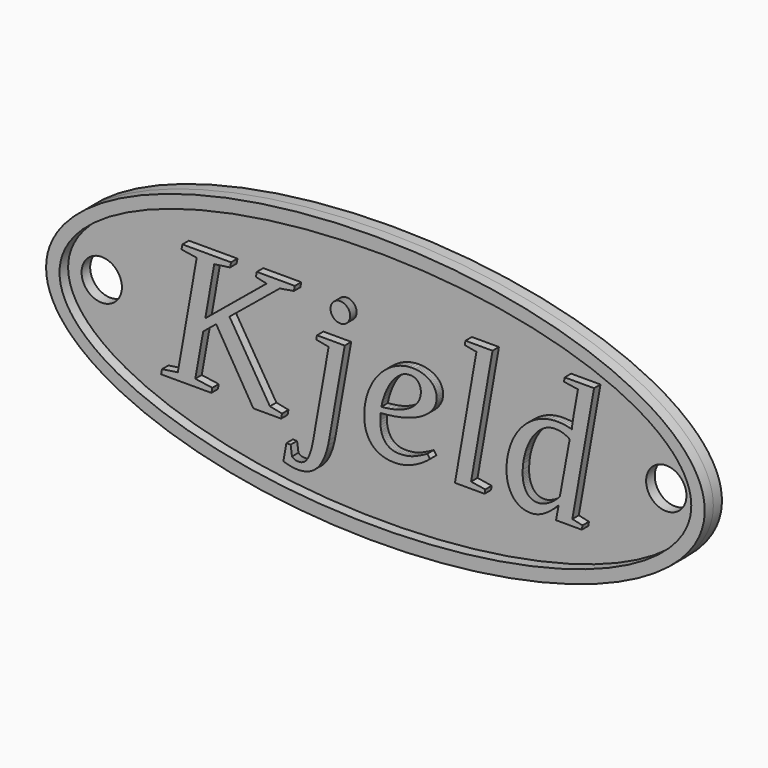
from build123d import *

# Parameters (mm, degrees)
F0_R     = 3
F1_DEPTH = 1.6
F2_DEPTH = 1.6
F3_DEPTH = 1.2


# Not quite as in the source:
# - a feature names something its author has since deleted; it is built from what else it names


with BuildPart() as f1:
    # F0 (on Front) → F1 (new body)
    with BuildSketch(Plane.XZ):
        with BuildLine():
            add(Edge.make_bspline(
                [(49, 0), (49, 34.6410161514), (-24.5, 17.3205080757), (-98, 0), (-24.5, -17.3205080757), (49, -34.6410161514), (49, 0)],
                knots=[0, 0, 0, 2.0943951024, 2.0943951024, 4.1887902048, 4.1887902048, 6.2831853072, 6.2831853072, 6.2831853072], degree=2, weights=[1, 0.5, 1, 0.5, 1, 0.5, 1]))
        make_face()
        with BuildLine():
            add(Edge.make_bspline(
                [(47, 0), (47, 31.1769145362), (-23.5, 15.5884572681), (-94, 0), (-23.5, -15.5884572681), (47, -31.1769145362), (47, 0)],
                knots=[0, 0, 0, 2.0943951024, 2.0943951024, 4.1887902048, 4.1887902048, 6.2831853072, 6.2831853072, 6.2831853072], degree=2, weights=[1, 0.5, 1, 0.5, 1, 0.5, 1]))
        make_face(mode=Mode.SUBTRACT)
        with BuildLine():
            add(Edge.make_bspline(
                [(47, 0), (47, 31.1769145362), (-23.5, 15.5884572681), (-94, 0), (-23.5, -15.5884572681), (47, -31.1769145362), (47, 0)],
                knots=[0, 0, 0, 2.0943951024, 2.0943951024, 4.1887902048, 4.1887902048, 6.2831853072, 6.2831853072, 6.2831853072], degree=2, weights=[1, 0.5, 1, 0.5, 1, 0.5, 1]))
        make_face()
        Polygon((-4.88085, 3.9466265909), (-7.22335, -9.2331734091), (-7.36215, -9.9206734091), (-7.52285, -10.5558734091), (-7.61145, -10.8539734091), (-7.70545, -11.1389734091), (-7.80495, -11.4109734091), (-7.90995, -11.6699734091), (-8.01705, -11.9198734091), (-8.12955, -12.1579734091), (-8.24755, -12.3842734091), (-8.37105, -12.5988734091), (-8.49995, -12.8016734091), (-8.63435, -12.9926734091), (-8.77425, -13.1718734091), (-8.91965, -13.3392734091), (-9.06685, -13.4953734091), (-9.21915, -13.6405734091), (-9.37655, -13.7747734091), (-9.53895, -13.8979734091), (-9.70635, -14.0103734091), (-9.87885, -14.1116734091), (-10.05635, -14.2021734091), (-10.23895, -14.2816734091), (-10.42615, -14.3510734091), (-10.61755, -14.4112734091), (-10.81325, -14.4621734091), (-11.01305, -14.5037734091), (-11.21705, -14.5361734091), (-11.42535, -14.5593734091), (-11.63785, -14.5732734091), (-11.85445, -14.5778734091), (-12.15565, -14.5694734091), (-12.45355, -14.5441734091), (-12.74805, -14.5021734091), (-13.03915, -14.4432734091), (-13.31685, -14.3809734091), (-13.44685, -14.3485734091), (-13.57095, -14.3153734091), (-13.68915, -14.2812734091), (-13.80145, -14.2463734091), (-13.90795, -14.2105734091), (-14.00845, -14.1739734091), (-13.56425, -11.6564734091), (-12.93145, -11.6564734091), (-12.72955, -13.1373734091), (-12.69125, -13.1737734091), (-12.65045, -13.2088734091), (-12.60715, -13.2427734091), (-12.56125, -13.2753734091), (-12.51285, -13.3066734091), (-12.46195, -13.3367734091), (-12.40855, -13.3655734091), (-12.35255, -13.3931734091), (-12.29345, -13.4183734091), (-12.23055, -13.4402734091), (-12.16385, -13.4587734091), (-12.09345, -13.4739734091), (-12.01915, -13.4856734091), (-11.94115, -13.4940734091), (-11.85935, -13.4991734091), (-11.77365, -13.5008734091), (-11.68025, -13.4983734091), (-11.58855, -13.4907734091), (-11.49855, -13.4781734091), (-11.41025, -13.4604734091), (-11.32355, -13.4377734091), (-11.23855, -13.4099734091), (-11.15525, -13.3771734091), (-11.07365, -13.3392734091), (-10.99375, -13.2951734091), (-10.91545, -13.2433734091), (-10.83885, -13.1840734091), (-10.76395, -13.1171734091), (-10.69075, -13.0426734091), (-10.61925, -12.9606734091), (-10.54945, -12.8710734091), (-10.48125, -12.7738734091), (-10.41465, -12.6682734091), (-10.34915, -12.5533734091), (-10.28505, -12.4292734091), (-10.22215, -12.2959734091), (-10.16045, -12.1533734091), (-10.10015, -12.0014734091), (-10.04105, -11.8403734091), (-9.98315, -11.6699734091), (-9.92655, -11.4923734091), (-9.87125, -11.3030734091), (-9.81725, -11.1019734091), (-9.76445, -10.8890734091), (-9.71285, -10.6644734091), (-9.66255, -10.4279734091), (-9.61355, -10.1797734091), (-9.56585, -9.9197734091), (-7.27715, 3.0042265909), (-9.12155, 3.3408265909), (-9.01385, 3.9466265909), align=None, mode=Mode.SUBTRACT)
        Polygon((8.79375, 1.6700265909), (8.79775, 1.5234265909), (8.78915, 1.3061265909), (8.76325, 1.0917265909), (8.72015, 0.8803265909), (8.65985, 0.6718265909), (8.58215, 0.4663265909), (8.48735, 0.2638265909), (8.37515, 0.0641265909), (8.24585, -0.1324734091), (8.09985, -0.3253734091), (7.93785, -0.5136734091), (7.75995, -0.6972734091), (7.56595, -0.8762734091), (7.35605, -1.0506734091), (7.13015, -1.2204734091), (6.88825, -1.3855734091), (6.63035, -1.5460734091), (6.35985, -1.6979734091), (6.07335, -1.8439734091), (5.77085, -1.9840734091), (5.45235, -2.1182734091), (5.11785, -2.2465734091), (4.76745, -2.3689734091), (4.01855, -2.5961734091), (3.21585, -2.7871734091), (2.35595, -2.9428734091), (1.43885, -3.0631734091), (0.46445, -3.1481734091), (0.46275, -3.1637734091), (0.46085, -3.1805734091), (0.45895, -3.1982734091), (0.45685, -3.2171734091), (0.45475, -3.2369734091), (0.45245, -3.2579734091), (0.45015, -3.2798734091), (0.44765, -3.3029734091), (0.44235, -3.3521734091), (0.43665, -3.4055734091), (0.43055, -3.4632734091), (0.42405, -3.5250734091), (0.42095, -3.5904734091), (0.41585, -3.7301734091), (0.41255, -3.8816734091), (0.41085, -4.0448734091), (0.41065, -4.1308734091), (0.41815, -4.4581734091), (0.44095, -4.7804734091), (0.47875, -5.0976734091), (0.53175, -5.4098734091), (0.56835, -5.5625734091), (0.61085, -5.7110734091), (0.65925, -5.8553734091), (0.71355, -5.9954734091), (0.77365, -6.1313734091), (0.83975, -6.2630734091), (0.91165, -6.3904734091), (0.98955, -6.5137734091), (1.07385, -6.6319734091), (1.16535, -6.7442734091), (1.26405, -6.8507734091), (1.36985, -6.9512734091), (1.48275, -7.0459734091), (1.60285, -7.1347734091), (1.73015, -7.2175734091), (1.86455, -7.2945734091), (2.00715, -7.3608734091), (2.15905, -7.4182734091), (2.32015, -7.4668734091), (2.49055, -7.5066734091), (2.67025, -7.5375734091), (2.85915, -7.5596734091), (3.05725, -7.5728734091), (3.26465, -7.5772734091), (3.56465, -7.5709734091), (3.85875, -7.5520734091), (4.14685, -7.5204734091), (4.42915, -7.4763734091), (4.70555, -7.4195734091), (4.97615, -7.3501734091), (5.24075, -7.2680734091), (5.49945, -7.1734734091), (6.00265, -6.9580734091), (6.95845, -6.4868734091), (7.41115, -6.2310734091), (7.80155, -6.7964734091), (7.57695, -6.9798734091), (7.33375, -7.1666734091), (7.07205, -7.3568734091), (6.79185, -7.5503734091), (6.49565, -7.7413734091), (6.18605, -7.9239734091), (5.52635, -8.2638734091), (5.18475, -8.4119734091), (4.83305, -8.5465734091), (4.47125, -8.6677734091), (4.09935, -8.7754734091), (3.72075, -8.8638734091), (3.33875, -8.9269734091), (2.95335, -8.9647734091), (2.56465, -8.9774734091), (2.28315, -8.9723734091), (2.01095, -8.9572734091), (1.74805, -8.9319734091), (1.49435, -8.8966734091), (1.24995, -8.8511734091), (1.01475, -8.7956734091), (0.78885, -8.7300734091), (0.57215, -8.6543734091), (0.36455, -8.5659734091), (0.16575, -8.4691734091), (-0.02415, -8.3640734091), (-0.20535, -8.2504734091), (-0.37755, -8.1284734091), (-0.54105, -7.9980734091), (-0.69565, -7.8591734091), (-0.84145, -7.7119734091), (-0.97835, -7.5562734091), (-1.10645, -7.3921734091), (-1.22575, -7.2196734091), (-1.33615, -7.0387734091), (-1.43775, -6.8494734091), (-1.53055, -6.6517734091), (-1.61445, -6.4455734091), (-1.68955, -6.2310734091), (-1.75585, -6.0089734091), (-1.81325, -5.7800734091), (-1.86185, -5.5444734091), (-1.90155, -5.3021734091), (-1.93255, -5.0530734091), (-1.96785, -4.5347734091), (-1.97225, -4.2654734091), (-1.95545, -3.6731734091), (-1.90495, -3.0942734091), (-1.82085, -2.5288734091), (-1.70305, -1.9768734091), (-1.55495, -1.4349734091), (-1.37995, -0.9133734091), (-1.17795, -0.4118734091), (-0.94915, 0.0694265909), (-0.69505, 0.5355265909), (-0.41735, 0.9781265909), (-0.11615, 1.3971265909), (0.20865, 1.7926265909), (0.55195, 2.1687265909), (0.90875, 2.5162265909), (1.27895, 2.8351265909), (1.66265, 3.1254265909), (2.06485, 3.3854265909), (2.47715, 3.6134265909), (2.89955, 3.8095265909), (3.33195, 3.9735265909), (3.77795, 4.1090265909), (4.22725, 4.2058265909), (4.67995, 4.2638265909), (5.13595, 4.2832265909), (5.55495, 4.2697265909), (5.75565, 4.2529265909), (5.95045, 4.2293265909), (6.13935, 4.1990265909), (6.32235, 4.1620265909), (6.49945, 4.1183265909), (6.67075, 4.0678265909), (6.83895, 4.0146265909), (7.00055, 3.9559265909), (7.15535, 3.8917265909), (7.30345, 3.8221265909), (7.44485, 3.7470265909), (7.57945, 3.6664265909), (7.70735, 3.5804265909), (7.82845, 3.4889265909), (7.94275, 3.3957265909), (8.04975, 3.2979265909), (8.14965, 3.1955265909), (8.24245, 3.0884265909), (8.32805, 2.9767265909), (8.40655, 2.8604265909), (8.47785, 2.7394265909), (8.54205, 2.6138265909), (8.60195, 2.4878265909), (8.65395, 2.3589265909), (8.69785, 2.2270265909), (8.73385, 2.0922265909), (8.76185, 1.9544265909), (8.78185, 1.8136265909), align=None, mode=Mode.SUBTRACT)
        with Locations((-42, 0)):
            Circle(F0_R, mode=Mode.SUBTRACT)
        Polygon((-17.96715, 9.3451265909), (-12.31285, 9.3451265909), (-12.44745, 8.6316265909), (-14.54765, 8.2816265909), (-22.03285, 2.1561265909), (-16.01505, -7.6311734091), (-14.21105, -7.9946734091), (-14.34575, -8.7081734091), (-18.47875, -8.7081734091), (-24.01185, 0.5271265909), (-25.93695, -1.0479734091), (-27.12165, -7.6311734091), (-24.59075, -7.9946734091), (-24.72535, -8.7081734091), (-32.21055, -8.7081734091), (-32.07595, -7.9946734091), (-29.71995, -7.6311734091), (-26.90625, 8.2816265909), (-29.16805, 8.6316265909), (-29.03335, 9.3451265909), (-21.80395, 9.3451265909), (-21.93865, 8.6316265909), (-24.30805, 8.2816265909), (-25.62735, 0.7695265909), (-16.49975, 8.2816265909), (-18.10175, 8.6316265909), align=None, mode=Mode.SUBTRACT)
        Polygon((-4.07495, 8.1533265909), (-4.07305, 8.0796265909), (-4.07495, 8.0060265909), (-4.08065, 7.9332265909), (-4.09015, 7.8613265909), (-4.10335, 7.7902265909), (-4.12045, 7.7199265909), (-4.14125, 7.6505265909), (-4.16585, 7.5819265909), (-4.19425, 7.5142265909), (-4.22265, 7.4511265909), (-4.25405, 7.3897265909), (-4.28825, 7.3299265909), (-4.32555, 7.2719265909), (-4.36575, 7.2155265909), (-4.40885, 7.1608265909), (-4.45485, 7.1078265909), (-4.50395, 7.0565265909), (-4.55545, 7.0073265909), (-4.60905, 6.9606265909), (-4.66485, 6.9164265909), (-4.72265, 6.8747265909), (-4.78265, 6.8356265909), (-4.84465, 6.7990265909), (-4.90885, 6.7649265909), (-4.97505, 6.7334265909), (-5.04285, 6.7081265909), (-5.11145, 6.6863265909), (-5.18085, 6.6677265909), (-5.25105, 6.6526265909), (-5.32215, 6.6408265909), (-5.39415, 6.6324265909), (-5.46685, 6.6274265909), (-5.54055, 6.6257265909), (-5.61415, 6.6274265909), (-5.68695, 6.6324265909), (-5.75885, 6.6408265909), (-5.82995, 6.6526265909), (-5.90025, 6.6677265909), (-5.96965, 6.6863265909), (-6.03825, 6.7081265909), (-6.10595, 6.7334265909), (-6.23045, 6.7990265909), (-6.34825, 6.8747265909), (-6.45935, 6.9606265909), (-6.56365, 7.0565265909), (-6.65955, 7.1608265909), (-6.74545, 7.2719265909), (-6.82115, 7.3897265909), (-6.88675, 7.5142265909), (-6.91205, 7.5819265909), (-6.93385, 7.6505265909), (-6.95245, 7.7199265909), (-6.96755, 7.7902265909), (-6.97935, 7.8613265909), (-6.98775, 7.9332265909), (-6.99275, 8.0060265909), (-6.99445, 8.0796265909), (-6.99275, 8.1533265909), (-6.98775, 8.2260265909), (-6.97935, 8.2980265909), (-6.96755, 8.3691265909), (-6.95245, 8.4393265909), (-6.93385, 8.5087265909), (-6.91205, 8.5773265909), (-6.88675, 8.6451265909), (-6.85525, 8.7113265909), (-6.82115, 8.7755265909), (-6.78455, 8.8375265909), (-6.74545, 8.8975265909), (-6.70375, 8.9553265909), (-6.65955, 9.0111265909), (-6.61285, 9.0647265909), (-6.56365, 9.1162265909), (-6.51235, 9.1653265909), (-6.45935, 9.2113265909), (-6.40465, 9.2544265909), (-6.34825, 9.2946265909), (-6.29025, 9.3319265909), (-6.23045, 9.3661265909), (-6.16905, 9.3975265909), (-6.10595, 9.4259265909), (-6.03825, 9.4543265909), (-5.96965, 9.4789265909), (-5.90025, 9.4997265909), (-5.82995, 9.5168265909), (-5.75885, 9.5300265909), (-5.68695, 9.5395265909), (-5.61415, 9.5452265909), (-5.54055, 9.5470265909), (-5.46685, 9.5452265909), (-5.39415, 9.5395265909), (-5.32215, 9.5300265909), (-5.25105, 9.5168265909), (-5.18085, 9.4997265909), (-5.11145, 9.4789265909), (-5.04285, 9.4543265909), (-4.97505, 9.4259265909), (-4.90885, 9.3975265909), (-4.84465, 9.3661265909), (-4.78265, 9.3319265909), (-4.72265, 9.2946265909), (-4.66485, 9.2544265909), (-4.60905, 9.2113265909), (-4.55545, 9.1653265909), (-4.50395, 9.1162265909), (-4.45485, 9.0647265909), (-4.40885, 9.0111265909), (-4.36575, 8.9553265909), (-4.32555, 8.8975265909), (-4.28825, 8.8375265909), (-4.25405, 8.7755265909), (-4.22265, 8.7113265909), (-4.19425, 8.6451265909), (-4.16585, 8.5773265909), (-4.14125, 8.5087265909), (-4.12045, 8.4393265909), (-4.10335, 8.3691265909), (-4.09015, 8.2980265909), (-4.08065, 8.2260265909), align=None, mode=Mode.SUBTRACT)
        Polygon((17.10485, 10.4221265909), (13.91425, -7.7657734091), (16.02785, -8.1023734091), (15.92015, -8.7081734091), (11.51795, -8.7081734091), (14.70855, 9.4932265909), (12.97185, 9.8163265909), (13.07955, 10.4221265909), align=None, mode=Mode.SUBTRACT)
        Polygon((28.66405, 4.0299265909), (28.89875, 3.9601265909), (28.90055, 3.9808265909), (28.90255, 4.0026265909), (28.90475, 4.0254265909), (28.90715, 4.0493265909), (28.91265, 4.1002265909), (28.91895, 4.1553265909), (28.92615, 4.2146265909), (28.93415, 4.2781265909), (28.94295, 4.3459265909), (28.95265, 4.4178265909), (28.97365, 4.5735265909), (29.02075, 4.8898265909), (29.04685, 5.0505265909), (29.07295, 5.2171265909), (29.12005, 5.5403265909), (29.14105, 5.6968265909), (29.15435, 5.7725265909), (29.16715, 5.8448265909), (29.17955, 5.9138265909), (29.19155, 5.9795265909), (29.20315, 6.0417265909), (29.21425, 6.1006265909), (29.22505, 6.1562265909), (29.23535, 6.2083265909), (29.81425, 9.4932265909), (27.74095, 9.8163265909), (27.84865, 10.4221265909), (32.21055, 10.4221265909), (28.97955, -7.7657734091), (30.50085, -8.1023734091), (30.39315, -8.7081734091), (26.55625, -8.7081734091), (26.94665, -6.6079734091), (26.66545, -6.8951734091), (26.38715, -7.1641734091), (26.11175, -7.4151734091), (25.83935, -7.6479734091), (25.56995, -7.8627734091), (25.30345, -8.0594734091), (25.03985, -8.2380734091), (24.77925, -8.3985734091), (24.52135, -8.5373734091), (24.26595, -8.6576734091), (24.01315, -8.7594734091), (23.76275, -8.8427734091), (23.51495, -8.9075734091), (23.26975, -8.9538734091), (23.02695, -8.9816734091), (22.78675, -8.9908734091), (22.58715, -8.9860734091), (22.39215, -8.9715734091), (22.20175, -8.9473734091), (22.01605, -8.9134734091), (21.83495, -8.8699734091), (21.65845, -8.8166734091), (21.48655, -8.7537734091), (21.31935, -8.6812734091), (21.15735, -8.5996734091), (21.00125, -8.5095734091), (20.85105, -8.4111734091), (20.70675, -8.3042734091), (20.56835, -8.1889734091), (20.43585, -8.0653734091), (20.30925, -7.9332734091), (20.18845, -7.7926734091), (20.07385, -7.6406734091), (19.96555, -7.4805734091), (19.86345, -7.3124734091), (19.76775, -7.1363734091), (19.67835, -6.9523734091), (19.59525, -6.7602734091), (19.51855, -6.5602734091), (19.44805, -6.3521734091), (19.38805, -6.1367734091), (19.33615, -5.9146734091), (19.29215, -5.6858734091), (19.22825, -5.2078734091), (19.19625, -4.7030734091), (19.19225, -4.4405734091), (19.20825, -3.8658734091), (19.25615, -3.2995734091), (19.33615, -2.7417734091), (19.44805, -2.1922734091), (19.58935, -1.6487734091), (19.75765, -1.1219734091), (19.95285, -0.6120734091), (20.17505, -0.1190734091), (20.42235, 0.3546265909), (20.69335, 0.8065265909), (20.98785, 1.2364265909), (21.30585, 1.6445265909), (21.65255, 2.0341265909), (22.01935, 2.3951265909), (22.40645, 2.7274265909), (22.81365, 3.0312265909), (23.23945, 3.3105265909), (23.68205, 3.5562265909), (24.14145, 3.7682265909), (24.61765, 3.9466265909), (25.11495, 4.0880265909), (25.62395, 4.1889265909), (26.14485, 4.2495265909), (26.67745, 4.2697265909), (27.00555, 4.2647265909), (27.31695, 4.2495265909), (27.61145, 4.2243265909), (27.88905, 4.1889265909), (28.15915, 4.1443265909), (28.41745, 4.0913265909), align=None, mode=Mode.SUBTRACT)
        with Locations((42, 0)):
            Circle(F0_R, mode=Mode.SUBTRACT)
        Polygon((28.90055, 3.9808265909), (28.89875, 3.9601265909), (28.66405, 4.0299265909), (28.41745, 4.0913265909), (28.15915, 4.1443265909), (27.88905, 4.1889265909), (27.61145, 4.2243265909), (27.31695, 4.2495265909), (27.00555, 4.2647265909), (26.67745, 4.2697265909), (26.14485, 4.2495265909), (25.62395, 4.1889265909), (25.11495, 4.0880265909), (24.61765, 3.9466265909), (24.14145, 3.7682265909), (23.68205, 3.5562265909), (23.23945, 3.3105265909), (22.81365, 3.0312265909), (22.40645, 2.7274265909), (22.01935, 2.3951265909), (21.65255, 2.0341265909), (21.30585, 1.6445265909), (20.98785, 1.2364265909), (20.69335, 0.8065265909), (20.42235, 0.3546265909), (20.17505, -0.1190734091), (19.95285, -0.6120734091), (19.75765, -1.1219734091), (19.58935, -1.6487734091), (19.44805, -2.1922734091), (19.33615, -2.7417734091), (19.25615, -3.2995734091), (19.20825, -3.8658734091), (19.19225, -4.4405734091), (19.19625, -4.7030734091), (19.22825, -5.2078734091), (19.29215, -5.6858734091), (19.33615, -5.9146734091), (19.38805, -6.1367734091), (19.44805, -6.3521734091), (19.51855, -6.5602734091), (19.59525, -6.7602734091), (19.67835, -6.9523734091), (19.76775, -7.1363734091), (19.86345, -7.3124734091), (19.96555, -7.4805734091), (20.07385, -7.6406734091), (20.18845, -7.7926734091), (20.30925, -7.9332734091), (20.43585, -8.0653734091), (20.56835, -8.1889734091), (20.70675, -8.3042734091), (20.85105, -8.4111734091), (21.00125, -8.5095734091), (21.15735, -8.5996734091), (21.31935, -8.6812734091), (21.48655, -8.7537734091), (21.65845, -8.8166734091), (21.83495, -8.8699734091), (22.01605, -8.9134734091), (22.20175, -8.9473734091), (22.39215, -8.9715734091), (22.58715, -8.9860734091), (22.78675, -8.9908734091), (23.02695, -8.9816734091), (23.26975, -8.9538734091), (23.51495, -8.9075734091), (23.76275, -8.8427734091), (24.01315, -8.7594734091), (24.26595, -8.6576734091), (24.52135, -8.5373734091), (24.77925, -8.3985734091), (25.03985, -8.2380734091), (25.30345, -8.0594734091), (25.56995, -7.8627734091), (25.83935, -7.6479734091), (26.11175, -7.4151734091), (26.38715, -7.1641734091), (26.66545, -6.8951734091), (26.94665, -6.6079734091), (26.55625, -8.7081734091), (30.39315, -8.7081734091), (30.50085, -8.1023734091), (28.97955, -7.7657734091), (32.21055, 10.4221265909), (27.84865, 10.4221265909), (27.74095, 9.8163265909), (29.81425, 9.4932265909), (29.23535, 6.2083265909), (29.22505, 6.1562265909), (29.21425, 6.1006265909), (29.20315, 6.0417265909), (29.19155, 5.9795265909), (29.17955, 5.9138265909), (29.16715, 5.8448265909), (29.15435, 5.7725265909), (29.14105, 5.6968265909), (29.12005, 5.5403265909), (29.07295, 5.2171265909), (29.04685, 5.0505265909), (29.02075, 4.8898265909), (28.97365, 4.5735265909), (28.95265, 4.4178265909), (28.94295, 4.3459265909), (28.93415, 4.2781265909), (28.92615, 4.2146265909), (28.91895, 4.1553265909), (28.91265, 4.1002265909), (28.90715, 4.0493265909), (28.90475, 4.0254265909), (28.90255, 4.0026265909), align=None)
        Polygon((28.35185, 2.7064265909), (28.58915, 2.5600265909), (27.12175, -5.4367734091), (26.91535, -5.6527734091), (26.49635, -6.0482734091), (26.28365, -6.2276734091), (26.06885, -6.3949734091), (25.85205, -6.5499734091), (25.63305, -6.6927734091), (25.41195, -6.8233734091), (25.19505, -6.9369734091), (24.98195, -7.0354734091), (24.77265, -7.1187734091), (24.56715, -7.1868734091), (24.36545, -7.2398734091), (24.16755, -7.2777734091), (23.97335, -7.3004734091), (23.78295, -7.3080734091), (23.67885, -7.3053734091), (23.57515, -7.2971734091), (23.47185, -7.2834734091), (23.36905, -7.2642734091), (23.26655, -7.2396734091), (23.16455, -7.2095734091), (23.06295, -7.1740734091), (22.96175, -7.1330734091), (22.86545, -7.0861734091), (22.77165, -7.0329734091), (22.68035, -6.9733734091), (22.59155, -6.9075734091), (22.50535, -6.8353734091), (22.42155, -6.7569734091), (22.34035, -6.6721734091), (22.26175, -6.5810734091), (22.18935, -6.4803734091), (22.12035, -6.3732734091), (22.05475, -6.2598734091), (21.99245, -6.1401734091), (21.93355, -6.0141734091), (21.87805, -5.8818734091), (21.82585, -5.7432734091), (21.77705, -5.5982734091), (21.73285, -5.4430734091), (21.69465, -5.2802734091), (21.66225, -5.1098734091), (21.63575, -4.9318734091), (21.61505, -4.7463734091), (21.60035, -4.5532734091), (21.59155, -4.3525734091), (21.58855, -4.1443734091), (21.59785, -3.7126734091), (21.67185, -2.8443734091), (21.73665, -2.4076734091), (21.82585, -1.9734734091), (22.05475, -1.1253734091), (22.19435, -0.7113734091), (22.35005, -0.3075734091), (22.52085, 0.0829265909), (22.70685, 0.4598265909), (22.90795, 0.8233265909), (23.13005, 1.1683265909), (23.36565, 1.4897265909), (23.61475, 1.7876265909), (23.87725, 2.0619265909), (24.01335, 2.1929265909), (24.29435, 2.4336265909), (24.58715, 2.6456265909), (24.89175, 2.8290265909), (25.04845, 2.9100265909), (25.20815, 2.9826265909), (25.37075, 3.0455265909), (25.53625, 3.0987265909), (25.70475, 3.1422265909), (25.87625, 3.1761265909), (26.05055, 3.2003265909), (26.22795, 3.2148265909), (26.40815, 3.2196265909), (26.58315, 3.2169265909), (26.75145, 3.2087265909), (26.91305, 3.1950265909), (27.06785, 3.1759265909), (27.21595, 3.1513265909), (27.35725, 3.1212265909), (27.49195, 3.0856265909), (27.61985, 3.0446265909), (27.86715, 2.9487265909), (28.11125, 2.8360265909), align=None, mode=Mode.SUBTRACT)
        Polygon((-12.44745, 8.6316265909), (-12.31285, 9.3451265909), (-17.96715, 9.3451265909), (-18.10175, 8.6316265909), (-16.49975, 8.2816265909), (-25.62735, 0.7695265909), (-24.30805, 8.2816265909), (-21.93865, 8.6316265909), (-21.80395, 9.3451265909), (-29.03335, 9.3451265909), (-29.16805, 8.6316265909), (-26.90625, 8.2816265909), (-29.71995, -7.6311734091), (-32.07595, -7.9946734091), (-32.21055, -8.7081734091), (-24.72535, -8.7081734091), (-24.59075, -7.9946734091), (-27.12165, -7.6311734091), (-25.93695, -1.0479734091), (-24.01185, 0.5271265909), (-18.47875, -8.7081734091), (-14.34575, -8.7081734091), (-14.21105, -7.9946734091), (-16.01505, -7.6311734091), (-22.03285, 2.1561265909), (-14.54765, 8.2816265909), align=None)
        Polygon((8.78915, 1.3061265909), (8.79775, 1.5234265909), (8.79375, 1.6700265909), (8.78185, 1.8136265909), (8.76185, 1.9544265909), (8.73385, 2.0922265909), (8.69785, 2.2270265909), (8.65395, 2.3589265909), (8.60195, 2.4878265909), (8.54205, 2.6138265909), (8.47785, 2.7394265909), (8.40655, 2.8604265909), (8.32805, 2.9767265909), (8.24245, 3.0884265909), (8.14965, 3.1955265909), (8.04975, 3.2979265909), (7.94275, 3.3957265909), (7.82845, 3.4889265909), (7.70735, 3.5804265909), (7.57945, 3.6664265909), (7.44485, 3.7470265909), (7.30345, 3.8221265909), (7.15535, 3.8917265909), (7.00055, 3.9559265909), (6.83895, 4.0146265909), (6.67075, 4.0678265909), (6.49945, 4.1183265909), (6.32235, 4.1620265909), (6.13935, 4.1990265909), (5.95045, 4.2293265909), (5.75565, 4.2529265909), (5.55495, 4.2697265909), (5.13595, 4.2832265909), (4.67995, 4.2638265909), (4.22725, 4.2058265909), (3.77795, 4.1090265909), (3.33195, 3.9735265909), (2.89955, 3.8095265909), (2.47715, 3.6134265909), (2.06485, 3.3854265909), (1.66265, 3.1254265909), (1.27895, 2.8351265909), (0.90875, 2.5162265909), (0.55195, 2.1687265909), (0.20865, 1.7926265909), (-0.11615, 1.3971265909), (-0.41735, 0.9781265909), (-0.69505, 0.5355265909), (-0.94915, 0.0694265909), (-1.17795, -0.4118734091), (-1.37995, -0.9133734091), (-1.55495, -1.4349734091), (-1.70305, -1.9768734091), (-1.82085, -2.5288734091), (-1.90495, -3.0942734091), (-1.95545, -3.6731734091), (-1.97225, -4.2654734091), (-1.96785, -4.5347734091), (-1.93255, -5.0530734091), (-1.90155, -5.3021734091), (-1.86185, -5.5444734091), (-1.81325, -5.7800734091), (-1.75585, -6.0089734091), (-1.68955, -6.2310734091), (-1.61445, -6.4455734091), (-1.53055, -6.6517734091), (-1.43775, -6.8494734091), (-1.33615, -7.0387734091), (-1.22575, -7.2196734091), (-1.10645, -7.3921734091), (-0.97835, -7.5562734091), (-0.84145, -7.7119734091), (-0.69565, -7.8591734091), (-0.54105, -7.9980734091), (-0.37755, -8.1284734091), (-0.20535, -8.2504734091), (-0.02415, -8.3640734091), (0.16575, -8.4691734091), (0.36455, -8.5659734091), (0.57215, -8.6543734091), (0.78885, -8.7300734091), (1.01475, -8.7956734091), (1.24995, -8.8511734091), (1.49435, -8.8966734091), (1.74805, -8.9319734091), (2.01095, -8.9572734091), (2.28315, -8.9723734091), (2.56465, -8.9774734091), (2.95335, -8.9647734091), (3.33875, -8.9269734091), (3.72075, -8.8638734091), (4.09935, -8.7754734091), (4.47125, -8.6677734091), (4.83305, -8.5465734091), (5.18475, -8.4119734091), (5.52635, -8.2638734091), (6.18605, -7.9239734091), (6.49565, -7.7413734091), (6.79185, -7.5503734091), (7.07205, -7.3568734091), (7.33375, -7.1666734091), (7.57695, -6.9798734091), (7.80155, -6.7964734091), (7.41115, -6.2310734091), (6.95845, -6.4868734091), (6.00265, -6.9580734091), (5.49945, -7.1734734091), (5.24075, -7.2680734091), (4.97615, -7.3501734091), (4.70555, -7.4195734091), (4.42915, -7.4763734091), (4.14685, -7.5204734091), (3.85875, -7.5520734091), (3.56465, -7.5709734091), (3.26465, -7.5772734091), (3.05725, -7.5728734091), (2.85915, -7.5596734091), (2.67025, -7.5375734091), (2.49055, -7.5066734091), (2.32015, -7.4668734091), (2.15905, -7.4182734091), (2.00715, -7.3608734091), (1.86455, -7.2945734091), (1.73015, -7.2175734091), (1.60285, -7.1347734091), (1.48275, -7.0459734091), (1.36985, -6.9512734091), (1.26405, -6.8507734091), (1.16535, -6.7442734091), (1.07385, -6.6319734091), (0.98955, -6.5137734091), (0.91165, -6.3904734091), (0.83975, -6.2630734091), (0.77365, -6.1313734091), (0.71355, -5.9954734091), (0.65925, -5.8553734091), (0.61085, -5.7110734091), (0.56835, -5.5625734091), (0.53175, -5.4098734091), (0.47875, -5.0976734091), (0.44095, -4.7804734091), (0.41815, -4.4581734091), (0.41065, -4.1308734091), (0.41085, -4.0448734091), (0.41255, -3.8816734091), (0.41585, -3.7301734091), (0.42095, -3.5904734091), (0.42405, -3.5250734091), (0.43055, -3.4632734091), (0.43665, -3.4055734091), (0.44235, -3.3521734091), (0.44765, -3.3029734091), (0.45015, -3.2798734091), (0.45245, -3.2579734091), (0.45475, -3.2369734091), (0.45685, -3.2171734091), (0.45895, -3.1982734091), (0.46085, -3.1805734091), (0.46275, -3.1637734091), (0.46445, -3.1481734091), (1.43885, -3.0631734091), (2.35595, -2.9428734091), (3.21585, -2.7871734091), (4.01855, -2.5961734091), (4.76745, -2.3689734091), (5.11785, -2.2465734091), (5.45235, -2.1182734091), (5.77085, -1.9840734091), (6.07335, -1.8439734091), (6.35985, -1.6979734091), (6.63035, -1.5460734091), (6.88825, -1.3855734091), (7.13015, -1.2204734091), (7.35605, -1.0506734091), (7.56595, -0.8762734091), (7.75995, -0.6972734091), (7.93785, -0.5136734091), (8.09985, -0.3253734091), (8.24585, -0.1324734091), (8.37515, 0.0641265909), (8.48735, 0.2638265909), (8.58215, 0.4663265909), (8.65985, 0.6718265909), (8.72015, 0.8803265909), (8.76325, 1.0917265909), align=None)
        Polygon((1.28315, -2.2309734091), (0.57215, -2.2999734091), (0.67315, -1.8144734091), (0.80105, -1.3272734091), (0.95585, -0.8384734091), (1.13755, -0.3478734091), (1.34285, 0.1376265909), (1.56835, 0.5978265909), (1.81405, 1.0328265909), (2.07995, 1.4426265909), (2.22345, 1.6365265909), (2.52295, 1.9966265909), (2.67905, 2.1628265909), (2.83935, 2.3198265909), (3.00385, 2.4674265909), (3.17255, 2.6058265909), (3.34545, 2.7350265909), (3.52195, 2.8549265909), (3.70135, 2.9588265909), (3.88375, 3.0467265909), (4.06905, 3.1187265909), (4.25735, 3.1746265909), (4.44855, 3.2146265909), (4.64265, 3.2386265909), (4.83975, 3.2466265909), (4.93595, 3.2447265909), (5.02915, 3.2390265909), (5.11935, 3.2295265909), (5.20665, 3.2163265909), (5.29105, 3.1992265909), (5.37245, 3.1784265909), (5.45085, 3.1538265909), (5.52635, 3.1254265909), (5.59895, 3.0932265909), (5.66855, 3.0572265909), (5.73525, 3.0175265909), (5.79905, 2.9739265909), (5.85975, 2.9266265909), (5.91765, 2.8755265909), (5.97255, 2.8206265909), (6.02455, 2.7619265909), (6.07505, 2.7003265909), (6.12235, 2.6365265909), (6.16635, 2.5707265909), (6.20705, 2.5028265909), (6.24455, 2.4327265909), (6.27885, 2.3606265909), (6.30975, 2.2863265909), (6.33755, 2.2099265909), (6.36195, 2.1315265909), (6.38315, 2.0509265909), (6.40105, 1.9683265909), (6.41575, 1.8835265909), (6.42715, 1.7966265909), (6.43535, 1.7076265909), (6.44185, 1.5234265909), (6.43615, 1.3523265909), (6.41915, 1.1826265909), (6.39075, 1.0141265909), (6.35095, 0.8469265909), (6.29985, 0.6809265909), (6.23735, 0.5162265909), (6.16355, 0.3527265909), (6.07835, 0.1906265909), (5.98155, 0.0341265909), (5.87305, -0.1190734091), (5.75275, -0.2688734091), (5.62065, -0.4152734091), (5.47675, -0.5582734091), (5.32105, -0.6979734091), (5.15365, -0.8342734091), (4.97445, -0.9671734091), (4.78675, -1.0927734091), (4.58735, -1.2137734091), (4.37615, -1.3300734091), (4.15325, -1.4417734091), (3.91845, -1.5487734091), (3.67195, -1.6512734091), (3.41365, -1.7490734091), (3.14355, -1.8422734091), (2.86185, -1.9259734091), (2.56885, -2.0021734091), (1.94875, -2.1316734091), align=None, mode=Mode.SUBTRACT)
        Polygon((27.12175, -5.4367734091), (28.58915, 2.5600265909), (28.35185, 2.7064265909), (28.11125, 2.8360265909), (27.86715, 2.9487265909), (27.61985, 3.0446265909), (27.49195, 3.0856265909), (27.35725, 3.1212265909), (27.21595, 3.1513265909), (27.06785, 3.1759265909), (26.91305, 3.1950265909), (26.75145, 3.2087265909), (26.58315, 3.2169265909), (26.40815, 3.2196265909), (26.22795, 3.2148265909), (26.05055, 3.2003265909), (25.87625, 3.1761265909), (25.70475, 3.1422265909), (25.53625, 3.0987265909), (25.37075, 3.0455265909), (25.20815, 2.9826265909), (25.04845, 2.9100265909), (24.89175, 2.8290265909), (24.58715, 2.6456265909), (24.29435, 2.4336265909), (24.01335, 2.1929265909), (23.87725, 2.0619265909), (23.61475, 1.7876265909), (23.36565, 1.4897265909), (23.13005, 1.1683265909), (22.90795, 0.8233265909), (22.70685, 0.4598265909), (22.52085, 0.0829265909), (22.35005, -0.3075734091), (22.19435, -0.7113734091), (22.05475, -1.1253734091), (21.82585, -1.9734734091), (21.73665, -2.4076734091), (21.67185, -2.8443734091), (21.59785, -3.7126734091), (21.58855, -4.1443734091), (21.59155, -4.3525734091), (21.60035, -4.5532734091), (21.61505, -4.7463734091), (21.63575, -4.9318734091), (21.66225, -5.1098734091), (21.69465, -5.2802734091), (21.73285, -5.4430734091), (21.77705, -5.5982734091), (21.82585, -5.7432734091), (21.87805, -5.8818734091), (21.93355, -6.0141734091), (21.99245, -6.1401734091), (22.05475, -6.2598734091), (22.12035, -6.3732734091), (22.18935, -6.4803734091), (22.26175, -6.5810734091), (22.34035, -6.6721734091), (22.42155, -6.7569734091), (22.50535, -6.8353734091), (22.59155, -6.9075734091), (22.68035, -6.9733734091), (22.77165, -7.0329734091), (22.86545, -7.0861734091), (22.96175, -7.1330734091), (23.06295, -7.1740734091), (23.16455, -7.2095734091), (23.26655, -7.2396734091), (23.36905, -7.2642734091), (23.47185, -7.2834734091), (23.57515, -7.2971734091), (23.67885, -7.3053734091), (23.78295, -7.3080734091), (23.97335, -7.3004734091), (24.16755, -7.2777734091), (24.36545, -7.2398734091), (24.56715, -7.1868734091), (24.77265, -7.1187734091), (24.98195, -7.0354734091), (25.19505, -6.9369734091), (25.41195, -6.8233734091), (25.63305, -6.6927734091), (25.85205, -6.5499734091), (26.06885, -6.3949734091), (26.28365, -6.2276734091), (26.49635, -6.0482734091), (26.91535, -5.6527734091), align=None)
        Polygon((16.02785, -8.1023734091), (13.91425, -7.7657734091), (17.10485, 10.4221265909), (13.07955, 10.4221265909), (12.97185, 9.8163265909), (14.70855, 9.4932265909), (11.51795, -8.7081734091), (15.92015, -8.7081734091), align=None)
        Polygon((-7.36215, -9.9206734091), (-7.22335, -9.2331734091), (-4.88085, 3.9466265909), (-9.01385, 3.9466265909), (-9.12155, 3.3408265909), (-7.27715, 3.0042265909), (-9.56585, -9.9197734091), (-9.61355, -10.1797734091), (-9.66255, -10.4279734091), (-9.71285, -10.6644734091), (-9.76445, -10.8890734091), (-9.81725, -11.1019734091), (-9.87125, -11.3030734091), (-9.92655, -11.4923734091), (-9.98315, -11.6699734091), (-10.04105, -11.8403734091), (-10.10015, -12.0014734091), (-10.16045, -12.1533734091), (-10.22215, -12.2959734091), (-10.28505, -12.4292734091), (-10.34915, -12.5533734091), (-10.41465, -12.6682734091), (-10.48125, -12.7738734091), (-10.54945, -12.8710734091), (-10.61925, -12.9606734091), (-10.69075, -13.0426734091), (-10.76395, -13.1171734091), (-10.83885, -13.1840734091), (-10.91545, -13.2433734091), (-10.99375, -13.2951734091), (-11.07365, -13.3392734091), (-11.15525, -13.3771734091), (-11.23855, -13.4099734091), (-11.32355, -13.4377734091), (-11.41025, -13.4604734091), (-11.49855, -13.4781734091), (-11.58855, -13.4907734091), (-11.68025, -13.4983734091), (-11.77365, -13.5008734091), (-11.85935, -13.4991734091), (-11.94115, -13.4940734091), (-12.01915, -13.4856734091), (-12.09345, -13.4739734091), (-12.16385, -13.4587734091), (-12.23055, -13.4402734091), (-12.29345, -13.4183734091), (-12.35255, -13.3931734091), (-12.40855, -13.3655734091), (-12.46195, -13.3367734091), (-12.51285, -13.3066734091), (-12.56125, -13.2753734091), (-12.60715, -13.2427734091), (-12.65045, -13.2088734091), (-12.69125, -13.1737734091), (-12.72955, -13.1373734091), (-12.93145, -11.6564734091), (-13.56425, -11.6564734091), (-14.00845, -14.1739734091), (-13.90795, -14.2105734091), (-13.80145, -14.2463734091), (-13.68915, -14.2812734091), (-13.57095, -14.3153734091), (-13.44685, -14.3485734091), (-13.31685, -14.3809734091), (-13.03915, -14.4432734091), (-12.74805, -14.5021734091), (-12.45355, -14.5441734091), (-12.15565, -14.5694734091), (-11.85445, -14.5778734091), (-11.63785, -14.5732734091), (-11.42535, -14.5593734091), (-11.21705, -14.5361734091), (-11.01305, -14.5037734091), (-10.81325, -14.4621734091), (-10.61755, -14.4112734091), (-10.42615, -14.3510734091), (-10.23895, -14.2816734091), (-10.05635, -14.2021734091), (-9.87885, -14.1116734091), (-9.70635, -14.0103734091), (-9.53895, -13.8979734091), (-9.37655, -13.7747734091), (-9.21915, -13.6405734091), (-9.06685, -13.4953734091), (-8.91965, -13.3392734091), (-8.77425, -13.1718734091), (-8.63435, -12.9926734091), (-8.49995, -12.8016734091), (-8.37105, -12.5988734091), (-8.24755, -12.3842734091), (-8.12955, -12.1579734091), (-8.01705, -11.9198734091), (-7.90995, -11.6699734091), (-7.80495, -11.4109734091), (-7.70545, -11.1389734091), (-7.61145, -10.8539734091), (-7.52285, -10.5558734091), align=None)
        Polygon((0.67315, -1.8144734091), (0.57215, -2.2999734091), (1.28315, -2.2309734091), (1.94875, -2.1316734091), (2.56885, -2.0021734091), (2.86185, -1.9259734091), (3.14355, -1.8422734091), (3.41365, -1.7490734091), (3.67195, -1.6512734091), (3.91845, -1.5487734091), (4.15325, -1.4417734091), (4.37615, -1.3300734091), (4.58735, -1.2137734091), (4.78675, -1.0927734091), (4.97445, -0.9671734091), (5.15365, -0.8342734091), (5.32105, -0.6979734091), (5.47675, -0.5582734091), (5.62065, -0.4152734091), (5.75275, -0.2688734091), (5.87305, -0.1190734091), (5.98155, 0.0341265909), (6.07835, 0.1906265909), (6.16355, 0.3527265909), (6.23735, 0.5162265909), (6.29985, 0.6809265909), (6.35095, 0.8469265909), (6.39075, 1.0141265909), (6.41915, 1.1826265909), (6.43615, 1.3523265909), (6.44185, 1.5234265909), (6.43535, 1.7076265909), (6.42715, 1.7966265909), (6.41575, 1.8835265909), (6.40105, 1.9683265909), (6.38315, 2.0509265909), (6.36195, 2.1315265909), (6.33755, 2.2099265909), (6.30975, 2.2863265909), (6.27885, 2.3606265909), (6.24455, 2.4327265909), (6.20705, 2.5028265909), (6.16635, 2.5707265909), (6.12235, 2.6365265909), (6.07505, 2.7003265909), (6.02455, 2.7619265909), (5.97255, 2.8206265909), (5.91765, 2.8755265909), (5.85975, 2.9266265909), (5.79905, 2.9739265909), (5.73525, 3.0175265909), (5.66855, 3.0572265909), (5.59895, 3.0932265909), (5.52635, 3.1254265909), (5.45085, 3.1538265909), (5.37245, 3.1784265909), (5.29105, 3.1992265909), (5.20665, 3.2163265909), (5.11935, 3.2295265909), (5.02915, 3.2390265909), (4.93595, 3.2447265909), (4.83975, 3.2466265909), (4.64265, 3.2386265909), (4.44855, 3.2146265909), (4.25735, 3.1746265909), (4.06905, 3.1187265909), (3.88375, 3.0467265909), (3.70135, 2.9588265909), (3.52195, 2.8549265909), (3.34545, 2.7350265909), (3.17255, 2.6058265909), (3.00385, 2.4674265909), (2.83935, 2.3198265909), (2.67905, 2.1628265909), (2.52295, 1.9966265909), (2.22345, 1.6365265909), (2.07995, 1.4426265909), (1.81405, 1.0328265909), (1.56835, 0.5978265909), (1.34285, 0.1376265909), (1.13755, -0.3478734091), (0.95585, -0.8384734091), (0.80105, -1.3272734091), align=None)
        Polygon((-4.07495, 8.0060265909), (-4.07305, 8.0796265909), (-4.07495, 8.1533265909), (-4.08065, 8.2260265909), (-4.09015, 8.2980265909), (-4.10335, 8.3691265909), (-4.12045, 8.4393265909), (-4.14125, 8.5087265909), (-4.16585, 8.5773265909), (-4.19425, 8.6451265909), (-4.22265, 8.7113265909), (-4.25405, 8.7755265909), (-4.28825, 8.8375265909), (-4.32555, 8.8975265909), (-4.36575, 8.9553265909), (-4.40885, 9.0111265909), (-4.45485, 9.0647265909), (-4.50395, 9.1162265909), (-4.55545, 9.1653265909), (-4.60905, 9.2113265909), (-4.66485, 9.2544265909), (-4.72265, 9.2946265909), (-4.78265, 9.3319265909), (-4.84465, 9.3661265909), (-4.90885, 9.3975265909), (-4.97505, 9.4259265909), (-5.04285, 9.4543265909), (-5.11145, 9.4789265909), (-5.18085, 9.4997265909), (-5.25105, 9.5168265909), (-5.32215, 9.5300265909), (-5.39415, 9.5395265909), (-5.46685, 9.5452265909), (-5.54055, 9.5470265909), (-5.61415, 9.5452265909), (-5.68695, 9.5395265909), (-5.75885, 9.5300265909), (-5.82995, 9.5168265909), (-5.90025, 9.4997265909), (-5.96965, 9.4789265909), (-6.03825, 9.4543265909), (-6.10595, 9.4259265909), (-6.16905, 9.3975265909), (-6.23045, 9.3661265909), (-6.29025, 9.3319265909), (-6.34825, 9.2946265909), (-6.40465, 9.2544265909), (-6.45935, 9.2113265909), (-6.51235, 9.1653265909), (-6.56365, 9.1162265909), (-6.61285, 9.0647265909), (-6.65955, 9.0111265909), (-6.70375, 8.9553265909), (-6.74545, 8.8975265909), (-6.78455, 8.8375265909), (-6.82115, 8.7755265909), (-6.85525, 8.7113265909), (-6.88675, 8.6451265909), (-6.91205, 8.5773265909), (-6.93385, 8.5087265909), (-6.95245, 8.4393265909), (-6.96755, 8.3691265909), (-6.97935, 8.2980265909), (-6.98775, 8.2260265909), (-6.99275, 8.1533265909), (-6.99445, 8.0796265909), (-6.99275, 8.0060265909), (-6.98775, 7.9332265909), (-6.97935, 7.8613265909), (-6.96755, 7.7902265909), (-6.95245, 7.7199265909), (-6.93385, 7.6505265909), (-6.91205, 7.5819265909), (-6.88675, 7.5142265909), (-6.82115, 7.3897265909), (-6.74545, 7.2719265909), (-6.65955, 7.1608265909), (-6.56365, 7.0565265909), (-6.45935, 6.9606265909), (-6.34825, 6.8747265909), (-6.23045, 6.7990265909), (-6.10595, 6.7334265909), (-6.03825, 6.7081265909), (-5.96965, 6.6863265909), (-5.90025, 6.6677265909), (-5.82995, 6.6526265909), (-5.75885, 6.6408265909), (-5.68695, 6.6324265909), (-5.61415, 6.6274265909), (-5.54055, 6.6257265909), (-5.46685, 6.6274265909), (-5.39415, 6.6324265909), (-5.32215, 6.6408265909), (-5.25105, 6.6526265909), (-5.18085, 6.6677265909), (-5.11145, 6.6863265909), (-5.04285, 6.7081265909), (-4.97505, 6.7334265909), (-4.90885, 6.7649265909), (-4.84465, 6.7990265909), (-4.78265, 6.8356265909), (-4.72265, 6.8747265909), (-4.66485, 6.9164265909), (-4.60905, 6.9606265909), (-4.55545, 7.0073265909), (-4.50395, 7.0565265909), (-4.45485, 7.1078265909), (-4.40885, 7.1608265909), (-4.36575, 7.2155265909), (-4.32555, 7.2719265909), (-4.28825, 7.3299265909), (-4.25405, 7.3897265909), (-4.22265, 7.4511265909), (-4.19425, 7.5142265909), (-4.16585, 7.5819265909), (-4.14125, 7.6505265909), (-4.12045, 7.7199265909), (-4.10335, 7.7902265909), (-4.09015, 7.8613265909), (-4.08065, 7.9332265909), align=None)
    extrude(amount=-F1_DEPTH)

    # F0 (on Front) → F2 (join)
    with BuildSketch(Plane.XZ):
        with BuildLine():
            add(Edge.make_bspline(
                [(49, 0), (49, 34.6410161514), (-24.5, 17.3205080757), (-98, 0), (-24.5, -17.3205080757), (49, -34.6410161514), (49, 0)],
                knots=[0, 0, 0, 2.0943951024, 2.0943951024, 4.1887902048, 4.1887902048, 6.2831853072, 6.2831853072, 6.2831853072], degree=2, weights=[1, 0.5, 1, 0.5, 1, 0.5, 1]))
        make_face()
        with BuildLine():
            add(Edge.make_bspline(
                [(47, 0), (47, 31.1769145362), (-23.5, 15.5884572681), (-94, 0), (-23.5, -15.5884572681), (47, -31.1769145362), (47, 0)],
                knots=[0, 0, 0, 2.0943951024, 2.0943951024, 4.1887902048, 4.1887902048, 6.2831853072, 6.2831853072, 6.2831853072], degree=2, weights=[1, 0.5, 1, 0.5, 1, 0.5, 1]))
        make_face(mode=Mode.SUBTRACT)
    extrude(amount=F2_DEPTH)

    # F0 (on Front) → F3 (join)
    with BuildSketch(Plane.XZ):
        Polygon((-12.44745, 8.6316265909), (-12.31285, 9.3451265909), (-17.96715, 9.3451265909), (-18.10175, 8.6316265909), (-16.49975, 8.2816265909), (-25.62735, 0.7695265909), (-24.30805, 8.2816265909), (-21.93865, 8.6316265909), (-21.80395, 9.3451265909), (-29.03335, 9.3451265909), (-29.16805, 8.6316265909), (-26.90625, 8.2816265909), (-29.71995, -7.6311734091), (-32.07595, -7.9946734091), (-32.21055, -8.7081734091), (-24.72535, -8.7081734091), (-24.59075, -7.9946734091), (-27.12165, -7.6311734091), (-25.93695, -1.0479734091), (-24.01185, 0.5271265909), (-18.47875, -8.7081734091), (-14.34575, -8.7081734091), (-14.21105, -7.9946734091), (-16.01505, -7.6311734091), (-22.03285, 2.1561265909), (-14.54765, 8.2816265909), align=None)
        Polygon((-7.36215, -9.9206734091), (-7.22335, -9.2331734091), (-4.88085, 3.9466265909), (-9.01385, 3.9466265909), (-9.12155, 3.3408265909), (-7.27715, 3.0042265909), (-9.56585, -9.9197734091), (-9.61355, -10.1797734091), (-9.66255, -10.4279734091), (-9.71285, -10.6644734091), (-9.76445, -10.8890734091), (-9.81725, -11.1019734091), (-9.87125, -11.3030734091), (-9.92655, -11.4923734091), (-9.98315, -11.6699734091), (-10.04105, -11.8403734091), (-10.10015, -12.0014734091), (-10.16045, -12.1533734091), (-10.22215, -12.2959734091), (-10.28505, -12.4292734091), (-10.34915, -12.5533734091), (-10.41465, -12.6682734091), (-10.48125, -12.7738734091), (-10.54945, -12.8710734091), (-10.61925, -12.9606734091), (-10.69075, -13.0426734091), (-10.76395, -13.1171734091), (-10.83885, -13.1840734091), (-10.91545, -13.2433734091), (-10.99375, -13.2951734091), (-11.07365, -13.3392734091), (-11.15525, -13.3771734091), (-11.23855, -13.4099734091), (-11.32355, -13.4377734091), (-11.41025, -13.4604734091), (-11.49855, -13.4781734091), (-11.58855, -13.4907734091), (-11.68025, -13.4983734091), (-11.77365, -13.5008734091), (-11.85935, -13.4991734091), (-11.94115, -13.4940734091), (-12.01915, -13.4856734091), (-12.09345, -13.4739734091), (-12.16385, -13.4587734091), (-12.23055, -13.4402734091), (-12.29345, -13.4183734091), (-12.35255, -13.3931734091), (-12.40855, -13.3655734091), (-12.46195, -13.3367734091), (-12.51285, -13.3066734091), (-12.56125, -13.2753734091), (-12.60715, -13.2427734091), (-12.65045, -13.2088734091), (-12.69125, -13.1737734091), (-12.72955, -13.1373734091), (-12.93145, -11.6564734091), (-13.56425, -11.6564734091), (-14.00845, -14.1739734091), (-13.90795, -14.2105734091), (-13.80145, -14.2463734091), (-13.68915, -14.2812734091), (-13.57095, -14.3153734091), (-13.44685, -14.3485734091), (-13.31685, -14.3809734091), (-13.03915, -14.4432734091), (-12.74805, -14.5021734091), (-12.45355, -14.5441734091), (-12.15565, -14.5694734091), (-11.85445, -14.5778734091), (-11.63785, -14.5732734091), (-11.42535, -14.5593734091), (-11.21705, -14.5361734091), (-11.01305, -14.5037734091), (-10.81325, -14.4621734091), (-10.61755, -14.4112734091), (-10.42615, -14.3510734091), (-10.23895, -14.2816734091), (-10.05635, -14.2021734091), (-9.87885, -14.1116734091), (-9.70635, -14.0103734091), (-9.53895, -13.8979734091), (-9.37655, -13.7747734091), (-9.21915, -13.6405734091), (-9.06685, -13.4953734091), (-8.91965, -13.3392734091), (-8.77425, -13.1718734091), (-8.63435, -12.9926734091), (-8.49995, -12.8016734091), (-8.37105, -12.5988734091), (-8.24755, -12.3842734091), (-8.12955, -12.1579734091), (-8.01705, -11.9198734091), (-7.90995, -11.6699734091), (-7.80495, -11.4109734091), (-7.70545, -11.1389734091), (-7.61145, -10.8539734091), (-7.52285, -10.5558734091), align=None)
        Polygon((-4.07495, 8.0060265909), (-4.07305, 8.0796265909), (-4.07495, 8.1533265909), (-4.08065, 8.2260265909), (-4.09015, 8.2980265909), (-4.10335, 8.3691265909), (-4.12045, 8.4393265909), (-4.14125, 8.5087265909), (-4.16585, 8.5773265909), (-4.19425, 8.6451265909), (-4.22265, 8.7113265909), (-4.25405, 8.7755265909), (-4.28825, 8.8375265909), (-4.32555, 8.8975265909), (-4.36575, 8.9553265909), (-4.40885, 9.0111265909), (-4.45485, 9.0647265909), (-4.50395, 9.1162265909), (-4.55545, 9.1653265909), (-4.60905, 9.2113265909), (-4.66485, 9.2544265909), (-4.72265, 9.2946265909), (-4.78265, 9.3319265909), (-4.84465, 9.3661265909), (-4.90885, 9.3975265909), (-4.97505, 9.4259265909), (-5.04285, 9.4543265909), (-5.11145, 9.4789265909), (-5.18085, 9.4997265909), (-5.25105, 9.5168265909), (-5.32215, 9.5300265909), (-5.39415, 9.5395265909), (-5.46685, 9.5452265909), (-5.54055, 9.5470265909), (-5.61415, 9.5452265909), (-5.68695, 9.5395265909), (-5.75885, 9.5300265909), (-5.82995, 9.5168265909), (-5.90025, 9.4997265909), (-5.96965, 9.4789265909), (-6.03825, 9.4543265909), (-6.10595, 9.4259265909), (-6.16905, 9.3975265909), (-6.23045, 9.3661265909), (-6.29025, 9.3319265909), (-6.34825, 9.2946265909), (-6.40465, 9.2544265909), (-6.45935, 9.2113265909), (-6.51235, 9.1653265909), (-6.56365, 9.1162265909), (-6.61285, 9.0647265909), (-6.65955, 9.0111265909), (-6.70375, 8.9553265909), (-6.74545, 8.8975265909), (-6.78455, 8.8375265909), (-6.82115, 8.7755265909), (-6.85525, 8.7113265909), (-6.88675, 8.6451265909), (-6.91205, 8.5773265909), (-6.93385, 8.5087265909), (-6.95245, 8.4393265909), (-6.96755, 8.3691265909), (-6.97935, 8.2980265909), (-6.98775, 8.2260265909), (-6.99275, 8.1533265909), (-6.99445, 8.0796265909), (-6.99275, 8.0060265909), (-6.98775, 7.9332265909), (-6.97935, 7.8613265909), (-6.96755, 7.7902265909), (-6.95245, 7.7199265909), (-6.93385, 7.6505265909), (-6.91205, 7.5819265909), (-6.88675, 7.5142265909), (-6.82115, 7.3897265909), (-6.74545, 7.2719265909), (-6.65955, 7.1608265909), (-6.56365, 7.0565265909), (-6.45935, 6.9606265909), (-6.34825, 6.8747265909), (-6.23045, 6.7990265909), (-6.10595, 6.7334265909), (-6.03825, 6.7081265909), (-5.96965, 6.6863265909), (-5.90025, 6.6677265909), (-5.82995, 6.6526265909), (-5.75885, 6.6408265909), (-5.68695, 6.6324265909), (-5.61415, 6.6274265909), (-5.54055, 6.6257265909), (-5.46685, 6.6274265909), (-5.39415, 6.6324265909), (-5.32215, 6.6408265909), (-5.25105, 6.6526265909), (-5.18085, 6.6677265909), (-5.11145, 6.6863265909), (-5.04285, 6.7081265909), (-4.97505, 6.7334265909), (-4.90885, 6.7649265909), (-4.84465, 6.7990265909), (-4.78265, 6.8356265909), (-4.72265, 6.8747265909), (-4.66485, 6.9164265909), (-4.60905, 6.9606265909), (-4.55545, 7.0073265909), (-4.50395, 7.0565265909), (-4.45485, 7.1078265909), (-4.40885, 7.1608265909), (-4.36575, 7.2155265909), (-4.32555, 7.2719265909), (-4.28825, 7.3299265909), (-4.25405, 7.3897265909), (-4.22265, 7.4511265909), (-4.19425, 7.5142265909), (-4.16585, 7.5819265909), (-4.14125, 7.6505265909), (-4.12045, 7.7199265909), (-4.10335, 7.7902265909), (-4.09015, 7.8613265909), (-4.08065, 7.9332265909), align=None)
        Polygon((8.78915, 1.3061265909), (8.79775, 1.5234265909), (8.79375, 1.6700265909), (8.78185, 1.8136265909), (8.76185, 1.9544265909), (8.73385, 2.0922265909), (8.69785, 2.2270265909), (8.65395, 2.3589265909), (8.60195, 2.4878265909), (8.54205, 2.6138265909), (8.47785, 2.7394265909), (8.40655, 2.8604265909), (8.32805, 2.9767265909), (8.24245, 3.0884265909), (8.14965, 3.1955265909), (8.04975, 3.2979265909), (7.94275, 3.3957265909), (7.82845, 3.4889265909), (7.70735, 3.5804265909), (7.57945, 3.6664265909), (7.44485, 3.7470265909), (7.30345, 3.8221265909), (7.15535, 3.8917265909), (7.00055, 3.9559265909), (6.83895, 4.0146265909), (6.67075, 4.0678265909), (6.49945, 4.1183265909), (6.32235, 4.1620265909), (6.13935, 4.1990265909), (5.95045, 4.2293265909), (5.75565, 4.2529265909), (5.55495, 4.2697265909), (5.13595, 4.2832265909), (4.67995, 4.2638265909), (4.22725, 4.2058265909), (3.77795, 4.1090265909), (3.33195, 3.9735265909), (2.89955, 3.8095265909), (2.47715, 3.6134265909), (2.06485, 3.3854265909), (1.66265, 3.1254265909), (1.27895, 2.8351265909), (0.90875, 2.5162265909), (0.55195, 2.1687265909), (0.20865, 1.7926265909), (-0.11615, 1.3971265909), (-0.41735, 0.9781265909), (-0.69505, 0.5355265909), (-0.94915, 0.0694265909), (-1.17795, -0.4118734091), (-1.37995, -0.9133734091), (-1.55495, -1.4349734091), (-1.70305, -1.9768734091), (-1.82085, -2.5288734091), (-1.90495, -3.0942734091), (-1.95545, -3.6731734091), (-1.97225, -4.2654734091), (-1.96785, -4.5347734091), (-1.93255, -5.0530734091), (-1.90155, -5.3021734091), (-1.86185, -5.5444734091), (-1.81325, -5.7800734091), (-1.75585, -6.0089734091), (-1.68955, -6.2310734091), (-1.61445, -6.4455734091), (-1.53055, -6.6517734091), (-1.43775, -6.8494734091), (-1.33615, -7.0387734091), (-1.22575, -7.2196734091), (-1.10645, -7.3921734091), (-0.97835, -7.5562734091), (-0.84145, -7.7119734091), (-0.69565, -7.8591734091), (-0.54105, -7.9980734091), (-0.37755, -8.1284734091), (-0.20535, -8.2504734091), (-0.02415, -8.3640734091), (0.16575, -8.4691734091), (0.36455, -8.5659734091), (0.57215, -8.6543734091), (0.78885, -8.7300734091), (1.01475, -8.7956734091), (1.24995, -8.8511734091), (1.49435, -8.8966734091), (1.74805, -8.9319734091), (2.01095, -8.9572734091), (2.28315, -8.9723734091), (2.56465, -8.9774734091), (2.95335, -8.9647734091), (3.33875, -8.9269734091), (3.72075, -8.8638734091), (4.09935, -8.7754734091), (4.47125, -8.6677734091), (4.83305, -8.5465734091), (5.18475, -8.4119734091), (5.52635, -8.2638734091), (6.18605, -7.9239734091), (6.49565, -7.7413734091), (6.79185, -7.5503734091), (7.07205, -7.3568734091), (7.33375, -7.1666734091), (7.57695, -6.9798734091), (7.80155, -6.7964734091), (7.41115, -6.2310734091), (6.95845, -6.4868734091), (6.00265, -6.9580734091), (5.49945, -7.1734734091), (5.24075, -7.2680734091), (4.97615, -7.3501734091), (4.70555, -7.4195734091), (4.42915, -7.4763734091), (4.14685, -7.5204734091), (3.85875, -7.5520734091), (3.56465, -7.5709734091), (3.26465, -7.5772734091), (3.05725, -7.5728734091), (2.85915, -7.5596734091), (2.67025, -7.5375734091), (2.49055, -7.5066734091), (2.32015, -7.4668734091), (2.15905, -7.4182734091), (2.00715, -7.3608734091), (1.86455, -7.2945734091), (1.73015, -7.2175734091), (1.60285, -7.1347734091), (1.48275, -7.0459734091), (1.36985, -6.9512734091), (1.26405, -6.8507734091), (1.16535, -6.7442734091), (1.07385, -6.6319734091), (0.98955, -6.5137734091), (0.91165, -6.3904734091), (0.83975, -6.2630734091), (0.77365, -6.1313734091), (0.71355, -5.9954734091), (0.65925, -5.8553734091), (0.61085, -5.7110734091), (0.56835, -5.5625734091), (0.53175, -5.4098734091), (0.47875, -5.0976734091), (0.44095, -4.7804734091), (0.41815, -4.4581734091), (0.41065, -4.1308734091), (0.41085, -4.0448734091), (0.41255, -3.8816734091), (0.41585, -3.7301734091), (0.42095, -3.5904734091), (0.42405, -3.5250734091), (0.43055, -3.4632734091), (0.43665, -3.4055734091), (0.44235, -3.3521734091), (0.44765, -3.3029734091), (0.45015, -3.2798734091), (0.45245, -3.2579734091), (0.45475, -3.2369734091), (0.45685, -3.2171734091), (0.45895, -3.1982734091), (0.46085, -3.1805734091), (0.46275, -3.1637734091), (0.46445, -3.1481734091), (1.43885, -3.0631734091), (2.35595, -2.9428734091), (3.21585, -2.7871734091), (4.01855, -2.5961734091), (4.76745, -2.3689734091), (5.11785, -2.2465734091), (5.45235, -2.1182734091), (5.77085, -1.9840734091), (6.07335, -1.8439734091), (6.35985, -1.6979734091), (6.63035, -1.5460734091), (6.88825, -1.3855734091), (7.13015, -1.2204734091), (7.35605, -1.0506734091), (7.56595, -0.8762734091), (7.75995, -0.6972734091), (7.93785, -0.5136734091), (8.09985, -0.3253734091), (8.24585, -0.1324734091), (8.37515, 0.0641265909), (8.48735, 0.2638265909), (8.58215, 0.4663265909), (8.65985, 0.6718265909), (8.72015, 0.8803265909), (8.76325, 1.0917265909), align=None)
        Polygon((1.28315, -2.2309734091), (0.57215, -2.2999734091), (0.67315, -1.8144734091), (0.80105, -1.3272734091), (0.95585, -0.8384734091), (1.13755, -0.3478734091), (1.34285, 0.1376265909), (1.56835, 0.5978265909), (1.81405, 1.0328265909), (2.07995, 1.4426265909), (2.22345, 1.6365265909), (2.52295, 1.9966265909), (2.67905, 2.1628265909), (2.83935, 2.3198265909), (3.00385, 2.4674265909), (3.17255, 2.6058265909), (3.34545, 2.7350265909), (3.52195, 2.8549265909), (3.70135, 2.9588265909), (3.88375, 3.0467265909), (4.06905, 3.1187265909), (4.25735, 3.1746265909), (4.44855, 3.2146265909), (4.64265, 3.2386265909), (4.83975, 3.2466265909), (4.93595, 3.2447265909), (5.02915, 3.2390265909), (5.11935, 3.2295265909), (5.20665, 3.2163265909), (5.29105, 3.1992265909), (5.37245, 3.1784265909), (5.45085, 3.1538265909), (5.52635, 3.1254265909), (5.59895, 3.0932265909), (5.66855, 3.0572265909), (5.73525, 3.0175265909), (5.79905, 2.9739265909), (5.85975, 2.9266265909), (5.91765, 2.8755265909), (5.97255, 2.8206265909), (6.02455, 2.7619265909), (6.07505, 2.7003265909), (6.12235, 2.6365265909), (6.16635, 2.5707265909), (6.20705, 2.5028265909), (6.24455, 2.4327265909), (6.27885, 2.3606265909), (6.30975, 2.2863265909), (6.33755, 2.2099265909), (6.36195, 2.1315265909), (6.38315, 2.0509265909), (6.40105, 1.9683265909), (6.41575, 1.8835265909), (6.42715, 1.7966265909), (6.43535, 1.7076265909), (6.44185, 1.5234265909), (6.43615, 1.3523265909), (6.41915, 1.1826265909), (6.39075, 1.0141265909), (6.35095, 0.8469265909), (6.29985, 0.6809265909), (6.23735, 0.5162265909), (6.16355, 0.3527265909), (6.07835, 0.1906265909), (5.98155, 0.0341265909), (5.87305, -0.1190734091), (5.75275, -0.2688734091), (5.62065, -0.4152734091), (5.47675, -0.5582734091), (5.32105, -0.6979734091), (5.15365, -0.8342734091), (4.97445, -0.9671734091), (4.78675, -1.0927734091), (4.58735, -1.2137734091), (4.37615, -1.3300734091), (4.15325, -1.4417734091), (3.91845, -1.5487734091), (3.67195, -1.6512734091), (3.41365, -1.7490734091), (3.14355, -1.8422734091), (2.86185, -1.9259734091), (2.56885, -2.0021734091), (1.94875, -2.1316734091), align=None, mode=Mode.SUBTRACT)
        Polygon((16.02785, -8.1023734091), (13.91425, -7.7657734091), (17.10485, 10.4221265909), (13.07955, 10.4221265909), (12.97185, 9.8163265909), (14.70855, 9.4932265909), (11.51795, -8.7081734091), (15.92015, -8.7081734091), align=None)
        Polygon((28.90055, 3.9808265909), (28.89875, 3.9601265909), (28.66405, 4.0299265909), (28.41745, 4.0913265909), (28.15915, 4.1443265909), (27.88905, 4.1889265909), (27.61145, 4.2243265909), (27.31695, 4.2495265909), (27.00555, 4.2647265909), (26.67745, 4.2697265909), (26.14485, 4.2495265909), (25.62395, 4.1889265909), (25.11495, 4.0880265909), (24.61765, 3.9466265909), (24.14145, 3.7682265909), (23.68205, 3.5562265909), (23.23945, 3.3105265909), (22.81365, 3.0312265909), (22.40645, 2.7274265909), (22.01935, 2.3951265909), (21.65255, 2.0341265909), (21.30585, 1.6445265909), (20.98785, 1.2364265909), (20.69335, 0.8065265909), (20.42235, 0.3546265909), (20.17505, -0.1190734091), (19.95285, -0.6120734091), (19.75765, -1.1219734091), (19.58935, -1.6487734091), (19.44805, -2.1922734091), (19.33615, -2.7417734091), (19.25615, -3.2995734091), (19.20825, -3.8658734091), (19.19225, -4.4405734091), (19.19625, -4.7030734091), (19.22825, -5.2078734091), (19.29215, -5.6858734091), (19.33615, -5.9146734091), (19.38805, -6.1367734091), (19.44805, -6.3521734091), (19.51855, -6.5602734091), (19.59525, -6.7602734091), (19.67835, -6.9523734091), (19.76775, -7.1363734091), (19.86345, -7.3124734091), (19.96555, -7.4805734091), (20.07385, -7.6406734091), (20.18845, -7.7926734091), (20.30925, -7.9332734091), (20.43585, -8.0653734091), (20.56835, -8.1889734091), (20.70675, -8.3042734091), (20.85105, -8.4111734091), (21.00125, -8.5095734091), (21.15735, -8.5996734091), (21.31935, -8.6812734091), (21.48655, -8.7537734091), (21.65845, -8.8166734091), (21.83495, -8.8699734091), (22.01605, -8.9134734091), (22.20175, -8.9473734091), (22.39215, -8.9715734091), (22.58715, -8.9860734091), (22.78675, -8.9908734091), (23.02695, -8.9816734091), (23.26975, -8.9538734091), (23.51495, -8.9075734091), (23.76275, -8.8427734091), (24.01315, -8.7594734091), (24.26595, -8.6576734091), (24.52135, -8.5373734091), (24.77925, -8.3985734091), (25.03985, -8.2380734091), (25.30345, -8.0594734091), (25.56995, -7.8627734091), (25.83935, -7.6479734091), (26.11175, -7.4151734091), (26.38715, -7.1641734091), (26.66545, -6.8951734091), (26.94665, -6.6079734091), (26.55625, -8.7081734091), (30.39315, -8.7081734091), (30.50085, -8.1023734091), (28.97955, -7.7657734091), (32.21055, 10.4221265909), (27.84865, 10.4221265909), (27.74095, 9.8163265909), (29.81425, 9.4932265909), (29.23535, 6.2083265909), (29.22505, 6.1562265909), (29.21425, 6.1006265909), (29.20315, 6.0417265909), (29.19155, 5.9795265909), (29.17955, 5.9138265909), (29.16715, 5.8448265909), (29.15435, 5.7725265909), (29.14105, 5.6968265909), (29.12005, 5.5403265909), (29.07295, 5.2171265909), (29.04685, 5.0505265909), (29.02075, 4.8898265909), (28.97365, 4.5735265909), (28.95265, 4.4178265909), (28.94295, 4.3459265909), (28.93415, 4.2781265909), (28.92615, 4.2146265909), (28.91895, 4.1553265909), (28.91265, 4.1002265909), (28.90715, 4.0493265909), (28.90475, 4.0254265909), (28.90255, 4.0026265909), align=None)
        Polygon((28.35185, 2.7064265909), (28.58915, 2.5600265909), (27.12175, -5.4367734091), (26.91535, -5.6527734091), (26.49635, -6.0482734091), (26.28365, -6.2276734091), (26.06885, -6.3949734091), (25.85205, -6.5499734091), (25.63305, -6.6927734091), (25.41195, -6.8233734091), (25.19505, -6.9369734091), (24.98195, -7.0354734091), (24.77265, -7.1187734091), (24.56715, -7.1868734091), (24.36545, -7.2398734091), (24.16755, -7.2777734091), (23.97335, -7.3004734091), (23.78295, -7.3080734091), (23.67885, -7.3053734091), (23.57515, -7.2971734091), (23.47185, -7.2834734091), (23.36905, -7.2642734091), (23.26655, -7.2396734091), (23.16455, -7.2095734091), (23.06295, -7.1740734091), (22.96175, -7.1330734091), (22.86545, -7.0861734091), (22.77165, -7.0329734091), (22.68035, -6.9733734091), (22.59155, -6.9075734091), (22.50535, -6.8353734091), (22.42155, -6.7569734091), (22.34035, -6.6721734091), (22.26175, -6.5810734091), (22.18935, -6.4803734091), (22.12035, -6.3732734091), (22.05475, -6.2598734091), (21.99245, -6.1401734091), (21.93355, -6.0141734091), (21.87805, -5.8818734091), (21.82585, -5.7432734091), (21.77705, -5.5982734091), (21.73285, -5.4430734091), (21.69465, -5.2802734091), (21.66225, -5.1098734091), (21.63575, -4.9318734091), (21.61505, -4.7463734091), (21.60035, -4.5532734091), (21.59155, -4.3525734091), (21.58855, -4.1443734091), (21.59785, -3.7126734091), (21.67185, -2.8443734091), (21.73665, -2.4076734091), (21.82585, -1.9734734091), (22.05475, -1.1253734091), (22.19435, -0.7113734091), (22.35005, -0.3075734091), (22.52085, 0.0829265909), (22.70685, 0.4598265909), (22.90795, 0.8233265909), (23.13005, 1.1683265909), (23.36565, 1.4897265909), (23.61475, 1.7876265909), (23.87725, 2.0619265909), (24.01335, 2.1929265909), (24.29435, 2.4336265909), (24.58715, 2.6456265909), (24.89175, 2.8290265909), (25.04845, 2.9100265909), (25.20815, 2.9826265909), (25.37075, 3.0455265909), (25.53625, 3.0987265909), (25.70475, 3.1422265909), (25.87625, 3.1761265909), (26.05055, 3.2003265909), (26.22795, 3.2148265909), (26.40815, 3.2196265909), (26.58315, 3.2169265909), (26.75145, 3.2087265909), (26.91305, 3.1950265909), (27.06785, 3.1759265909), (27.21595, 3.1513265909), (27.35725, 3.1212265909), (27.49195, 3.0856265909), (27.61985, 3.0446265909), (27.86715, 2.9487265909), (28.11125, 2.8360265909), align=None, mode=Mode.SUBTRACT)
    extrude(amount=F3_DEPTH)


solid = f1.part
